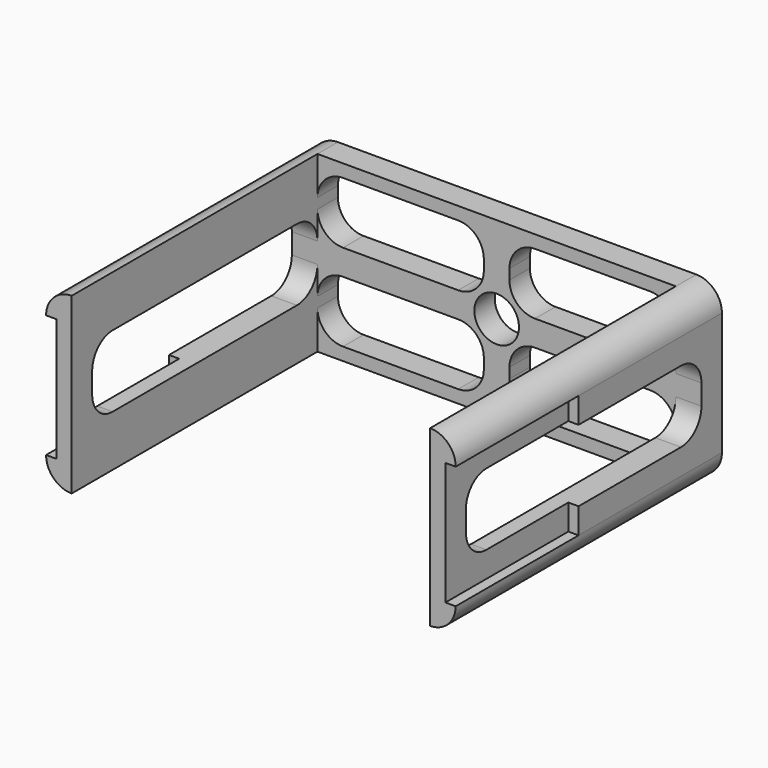
from build123d import *

# Parameters (mm, degrees)
F1_DEPTH  = 10
F2_R      = 8.7132034356
F3_DEPTH  = 11
F4_DEPTH  = 11
F6_DEPTH  = 120
F7_W      = 60
F7_H      = 48
F8_DEPTH  = 4
F10_DEPTH = 10


# Not quite as in the source:
# - a pattern or mirror of a feature is missing from the dataset's text; its kind, count and spacing are read off the source's solid


with BuildPart() as f1:
    # F0 (on Front) → F1 (new body)
    with BuildSketch(Plane.XZ):
        with BuildLine():
            Line((-70, -34), (70, -34))
            ThreePointArc((70, -34), (77.0710678119, -31.0710678119), (80, -24))
            Line((80, -24), (80, 24))
            ThreePointArc((80, 24), (77.0710678119, 31.0710678119), (70, 34))
            Line((70, 34), (-70, 34))
            ThreePointArc((-70, 34), (-77.0710678119, 31.0710678119), (-80, 24))
            Line((-80, 24), (-80, -24))
            ThreePointArc((-80, -24), (-77.0710678119, -31.0710678119), (-70, -34))
        make_face()
    extrude(amount=F1_DEPTH)

    # F2 (on face) → F3 (cut)
    with BuildSketch(Plane.XZ.offset(10)):
        with BuildLine():
            Line((15, 5), (60, 5))
            ThreePointArc((60, 5), (67.0710678119, 7.9289321881), (70, 15))
            Line((70, 15), (70, 19))
            ThreePointArc((70, 19), (67.0710678119, 26.0710678119), (60, 29))
            Line((60, 29), (15, 29))
            ThreePointArc((15, 29), (7.9289321881, 26.0710678119), (5, 19))
            Line((5, 19), (5, 15))
            ThreePointArc((5, 15), (7.9289321881, 7.9289321881), (15, 5))
        make_face()
        with BuildLine():
            ThreePointArc((70, -15), (67.0710678119, -7.9289321881), (60, -5))
            Line((60, -5), (15, -5))
            ThreePointArc((15, -5), (7.9289321881, -7.9289321881), (5, -15))
            Line((5, -15), (5, -19))
            ThreePointArc((5, -19), (7.9289321881, -26.0710678119), (15, -29))
            Line((15, -29), (60, -29))
            ThreePointArc((60, -29), (67.0710678119, -26.0710678119), (70, -19))
            Line((70, -19), (70, -15))
        make_face()
        with BuildLine():
            Line((-15, -5), (-60, -5))
            ThreePointArc((-60, -5), (-67.0710678119, -7.9289321881), (-70, -15))
            Line((-70, -15), (-70, -19))
            ThreePointArc((-70, -19), (-67.0710678119, -26.0710678119), (-60, -29))
            Line((-60, -29), (-15, -29))
            ThreePointArc((-15, -29), (-7.9289321881, -26.0710678119), (-5, -19))
            Line((-5, -19), (-5, -15))
            ThreePointArc((-5, -15), (-7.9289321881, -7.9289321881), (-15, -5))
        make_face()
        with BuildLine():
            ThreePointArc((-5, 19), (-7.9289321881, 26.0710678119), (-15, 29))
            Line((-15, 29), (-60, 29))
            ThreePointArc((-60, 29), (-67.0710678119, 26.0710678119), (-70, 19))
            Line((-70, 19), (-70, 15))
            ThreePointArc((-70, 15), (-67.0710678119, 7.9289321881), (-60, 5))
            Line((-60, 5), (-15, 5))
            ThreePointArc((-15, 5), (-7.9289321881, 7.9289321881), (-5, 15))
            Line((-5, 15), (-5, 19))
        make_face()
        Circle(F2_R)
    extrude(amount=-F3_DEPTH, mode=Mode.SUBTRACT)

    # F2 (on face) → F4 (cut)
    with BuildSketch(Plane.XZ.offset(10)):
        with BuildLine():
            Line((15, 5), (60, 5))
            ThreePointArc((60, 5), (67.0710678119, 7.9289321881), (70, 15))
            Line((70, 15), (70, 19))
            ThreePointArc((70, 19), (67.0710678119, 26.0710678119), (60, 29))
            Line((60, 29), (15, 29))
            ThreePointArc((15, 29), (7.9289321881, 26.0710678119), (5, 19))
            Line((5, 19), (5, 15))
            ThreePointArc((5, 15), (7.9289321881, 7.9289321881), (15, 5))
        make_face()
        with BuildLine():
            ThreePointArc((70, -15), (67.0710678119, -7.9289321881), (60, -5))
            Line((60, -5), (15, -5))
            ThreePointArc((15, -5), (7.9289321881, -7.9289321881), (5, -15))
            Line((5, -15), (5, -19))
            ThreePointArc((5, -19), (7.9289321881, -26.0710678119), (15, -29))
            Line((15, -29), (60, -29))
            ThreePointArc((60, -29), (67.0710678119, -26.0710678119), (70, -19))
            Line((70, -19), (70, -15))
        make_face()
        with BuildLine():
            Line((-15, -5), (-60, -5))
            ThreePointArc((-60, -5), (-67.0710678119, -7.9289321881), (-70, -15))
            Line((-70, -15), (-70, -19))
            ThreePointArc((-70, -19), (-67.0710678119, -26.0710678119), (-60, -29))
            Line((-60, -29), (-15, -29))
            ThreePointArc((-15, -29), (-7.9289321881, -26.0710678119), (-5, -19))
            Line((-5, -19), (-5, -15))
            ThreePointArc((-5, -15), (-7.9289321881, -7.9289321881), (-15, -5))
        make_face()
        with BuildLine():
            ThreePointArc((-5, 19), (-7.9289321881, 26.0710678119), (-15, 29))
            Line((-15, 29), (-60, 29))
            ThreePointArc((-60, 29), (-67.0710678119, 26.0710678119), (-70, 19))
            Line((-70, 19), (-70, 15))
            ThreePointArc((-70, 15), (-67.0710678119, 7.9289321881), (-60, 5))
            Line((-60, 5), (-15, 5))
            ThreePointArc((-15, 5), (-7.9289321881, 7.9289321881), (-5, 15))
            Line((-5, 15), (-5, 19))
        make_face()
        Circle(F2_R)
    extrude(amount=-F4_DEPTH, mode=Mode.SUBTRACT)

    # F5 (on face) → F6 (join)
    with BuildSketch(Plane.XZ.offset(10)):
        with BuildLine():
            Line((70, 34), (70, -34))
            ThreePointArc((70, -34), (77.0710678119, -31.0710678119), (80, -24))
            Line((80, -24), (80, 24))
            ThreePointArc((80, 24), (77.0710678119, 31.0710678119), (70, 34))
        make_face()
        with BuildLine():
            ThreePointArc((-80, -24), (-77.0710678119, -31.0710678119), (-70, -34))
            Line((-70, -34), (-70, 34))
            ThreePointArc((-70, 34), (-77.0710678119, 31.0710678119), (-80, 24))
            Line((-80, 24), (-80, -24))
        make_face()
    extrude(amount=F6_DEPTH)

    # F7 (on face) → F8 (cut)
    with BuildSketch(Plane(origin=(-80, 0, 0), x_dir=(0, -1, 0), z_dir=(-1, 0, 0))):
        with Locations((100, 0)):
            Rectangle(F7_W, F7_H)
    f8 = extrude(amount=-F8_DEPTH, mode=Mode.SUBTRACT)

    # F8_copies: F8 across plane
    add(f8.mirror(Plane(origin=(0, 0, 0), x_dir=(0, 0, 1), z_dir=(1, 0, 0))), mode=Mode.SUBTRACT)

    # F9 (on face) → F10 (cut)
    with BuildSketch(Plane(origin=(-80, 0, 0), x_dir=(0, -1, 0), z_dir=(-1, 0, 0))):
        with BuildLine():
            Line((20, -14), (110, -14))
            ThreePointArc((110, -14), (117.0710678119, -11.0710678119), (120, -4))
            Line((120, -4), (120, 4))
            ThreePointArc((120, 4), (117.0710678119, 11.0710678119), (110, 14))
            Line((110, 14), (20, 14))
            ThreePointArc((20, 14), (12.9289321881, 11.0710678119), (10, 4))
            Line((10, 4), (10, -4))
            ThreePointArc((10, -4), (12.9289321881, -11.0710678119), (20, -14))
        make_face()
    f10 = extrude(amount=-F10_DEPTH, mode=Mode.SUBTRACT)

    # F10_copies: F10 across plane
    add(f10.mirror(Plane(origin=(0, 0, 0), x_dir=(0, 0, 1), z_dir=(1, 0, 0))), mode=Mode.SUBTRACT)


solid = f1.part
